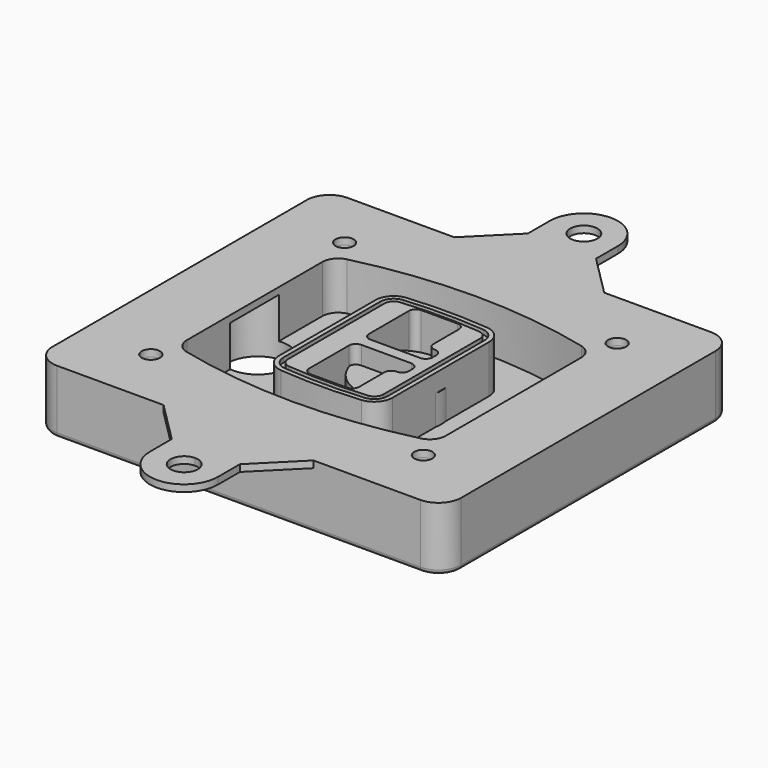
from build123d import *

# Parameters (mm, degrees)
F0_R      = 4
F1_DEPTH  = 25
F2_DEPTH  = 3
F3_DEPTH  = 18
F5_DEPTH  = 21
F6_DEPTH  = 2
F8_DEPTH  = 20
F9_DEPTH  = 16
F10_DEPTH = 25
F7_R      = 6
F7_R_2    = 4
F11_DEPTH = 6
F13_DEPTH = 9
F15_R     = 2
F16_R     = 4
F17_DEPTH = 3


# Not quite as in the source:
# - a feature of the source that left no trace in its solid (it failed there, or was rolled back) is left out
# - a feature names something its author has since deleted; it is built from what else it names


with BuildPart() as f1:
    # F0 (on Top) → F1 (new body)
    with BuildSketch(Plane.XY):
        with BuildLine():
            ThreePointArc((-90, -70), (-87.0710678119, -77.0710678119), (-80, -80))
            Line((-80, -80), (80, -80))
            ThreePointArc((80, -80), (87.0710678119, -77.0710678119), (90, -70))
            Line((90, -70), (90, 70))
            ThreePointArc((90, 70), (87.0710678119, 77.0710678119), (80, 80))
            Line((80, 80), (-80, 80))
            ThreePointArc((-80, 80), (-87.0710678119, 77.0710678119), (-90, 70))
            Line((-90, 70), (-90, -70))
        make_face()
        with Locations((-60, -53.3333333333)):
            Circle(F0_R, mode=Mode.SUBTRACT)
        with Locations((60, -53.3333333333)):
            Circle(F0_R, mode=Mode.SUBTRACT)
        with Locations((-60, 53.3333333333)):
            Circle(F0_R, mode=Mode.SUBTRACT)
        with BuildLine():
            ThreePointArc((-64, 37.2990447398), (-61.0143011354, 45.9411029726), (-53.3306899286, 50.8970778549))
            ThreePointArc((-53.3306899286, 50.8970778549), (0, 57.3333333333), (53.3306899286, 50.8970778549))
            ThreePointArc((53.3306899286, 50.8970778549), (61.0143011354, 45.9411029726), (64, 37.2990447398))
            Line((64, 37.2990447398), (64, -37.2990447398))
            ThreePointArc((64, -37.2990447398), (61.0143011354, -45.9411029726), (53.3306899286, -50.8970778549))
            ThreePointArc((53.3306899286, -50.8970778549), (0, -57.3333333333), (-53.3306899286, -50.8970778549))
            ThreePointArc((-53.3306899286, -50.8970778549), (-61.0143011354, -45.9411029726), (-64, -37.2990447398))
            Line((-64, -37.2990447398), (-64, 37.2990447398))
        make_face(mode=Mode.SUBTRACT)
        with Locations((60, 53.3333333333)):
            Circle(F0_R, mode=Mode.SUBTRACT)
        with BuildLine():
            ThreePointArc((53.3306899286, 50.8970778549), (0, 57.3333333333), (-53.3306899286, 50.8970778549))
            ThreePointArc((-53.3306899286, 50.8970778549), (-61.0143011354, 45.9411029726), (-64, 37.2990447398))
            Line((-64, 37.2990447398), (-64, -37.2990447398))
            ThreePointArc((-64, -37.2990447398), (-61.0143011354, -45.9411029726), (-53.3306899286, -50.8970778549))
            ThreePointArc((-53.3306899286, -50.8970778549), (0, -57.3333333333), (53.3306899286, -50.8970778549))
            ThreePointArc((53.3306899286, -50.8970778549), (61.0143011354, -45.9411029726), (64, -37.2990447398))
            Line((64, -37.2990447398), (64, 37.2990447398))
            ThreePointArc((64, 37.2990447398), (61.0143011354, 45.9411029726), (53.3306899286, 50.8970778549))
        make_face()
        with BuildLine():
            Line((-60, -37.2990447398), (-60, 37.2990447398))
            ThreePointArc((-60, 37.2990447398), (-57.8673579538, 43.4719434775), (-52.3790642347, 47.0119255363))
            ThreePointArc((-52.3790642347, 47.0119255363), (0, 53.3333333333), (52.3790642347, 47.0119255363))
            ThreePointArc((52.3790642347, 47.0119255363), (57.8673579538, 43.4719434775), (60, 37.2990447398))
            Line((60, 37.2990447398), (60, -37.2990447398))
            ThreePointArc((60, -37.2990447398), (57.8673579538, -43.4719434775), (52.3790642347, -47.0119255363))
            ThreePointArc((52.3790642347, -47.0119255363), (0, -53.3333333333), (-52.3790642347, -47.0119255363))
            ThreePointArc((-52.3790642347, -47.0119255363), (-57.8673579538, -43.4719434775), (-60, -37.2990447398))
        make_face(mode=Mode.SUBTRACT)
        with BuildLine():
            ThreePointArc((-52.3790642347, 47.0119255363), (-57.8673579538, 43.4719434775), (-60, 37.2990447398))
            Line((-60, 37.2990447398), (-60, -37.2990447398))
            ThreePointArc((-60, -37.2990447398), (-57.8673579538, -43.4719434775), (-52.3790642347, -47.0119255363))
            ThreePointArc((-52.3790642347, -47.0119255363), (0, -53.3333333333), (52.3790642347, -47.0119255363))
            ThreePointArc((52.3790642347, -47.0119255363), (57.8673579538, -43.4719434775), (60, -37.2990447398))
            Line((60, -37.2990447398), (60, 37.2990447398))
            ThreePointArc((60, 37.2990447398), (57.8673579538, 43.4719434775), (52.3790642347, 47.0119255363))
            ThreePointArc((52.3790642347, 47.0119255363), (0, 53.3333333333), (-52.3790642347, 47.0119255363))
        make_face()
        with BuildLine():
            ThreePointArc((51.6653449643, 44.0980612973), (55.5071505677, 41.6200738562), (57, 37.2990447398))
            Line((57, 37.2990447398), (57, -37.2990447398))
            ThreePointArc((57, -37.2990447398), (55.5071505677, -41.6200738562), (51.6653449643, -44.0980612973))
            ThreePointArc((51.6653449643, -44.0980612973), (0, -50.3333333333), (-51.6653449643, -44.0980612973))
            ThreePointArc((-51.6653449643, -44.0980612973), (-55.5071505677, -41.6200738562), (-57, -37.2990447398))
            Line((-57, -37.2990447398), (-57, 37.2990447398))
            ThreePointArc((-57, 37.2990447398), (-55.5071505677, 41.6200738562), (-51.6653449643, 44.0980612973))
            ThreePointArc((-51.6653449643, 44.0980612973), (0, 50.3333333333), (51.6653449643, 44.0980612973))
        make_face(mode=Mode.SUBTRACT)
        with BuildLine():
            Line((57, -37.2990447398), (57, 37.2990447398))
            ThreePointArc((57, 37.2990447398), (55.5071505677, 41.6200738562), (51.6653449643, 44.0980612973))
            ThreePointArc((51.6653449643, 44.0980612973), (0, 50.3333333333), (-51.6653449643, 44.0980612973))
            ThreePointArc((-51.6653449643, 44.0980612973), (-55.5071505677, 41.6200738562), (-57, 37.2990447398))
            Line((-57, 37.2990447398), (-57, -37.2990447398))
            ThreePointArc((-57, -37.2990447398), (-55.5071505677, -41.6200738562), (-51.6653449643, -44.0980612973))
            ThreePointArc((-51.6653449643, -44.0980612973), (0, -50.3333333333), (51.6653449643, -44.0980612973))
            ThreePointArc((51.6653449643, -44.0980612973), (55.5071505677, -41.6200738562), (57, -37.2990447398))
        make_face()
    extrude(amount=-F1_DEPTH)

    # F0 (on Top) → F2 (join)
    with BuildSketch(Plane.XY):
        with BuildLine():
            ThreePointArc((-52.3790642347, 47.0119255363), (-57.8673579538, 43.4719434775), (-60, 37.2990447398))
            Line((-60, 37.2990447398), (-60, -37.2990447398))
            ThreePointArc((-60, -37.2990447398), (-57.8673579538, -43.4719434775), (-52.3790642347, -47.0119255363))
            ThreePointArc((-52.3790642347, -47.0119255363), (0, -53.3333333333), (52.3790642347, -47.0119255363))
            ThreePointArc((52.3790642347, -47.0119255363), (57.8673579538, -43.4719434775), (60, -37.2990447398))
            Line((60, -37.2990447398), (60, 37.2990447398))
            ThreePointArc((60, 37.2990447398), (57.8673579538, 43.4719434775), (52.3790642347, 47.0119255363))
            ThreePointArc((52.3790642347, 47.0119255363), (0, 53.3333333333), (-52.3790642347, 47.0119255363))
        make_face()
        with BuildLine():
            ThreePointArc((51.6653449643, 44.0980612973), (55.5071505677, 41.6200738562), (57, 37.2990447398))
            Line((57, 37.2990447398), (57, -37.2990447398))
            ThreePointArc((57, -37.2990447398), (55.5071505677, -41.6200738562), (51.6653449643, -44.0980612973))
            ThreePointArc((51.6653449643, -44.0980612973), (0, -50.3333333333), (-51.6653449643, -44.0980612973))
            ThreePointArc((-51.6653449643, -44.0980612973), (-55.5071505677, -41.6200738562), (-57, -37.2990447398))
            Line((-57, -37.2990447398), (-57, 37.2990447398))
            ThreePointArc((-57, 37.2990447398), (-55.5071505677, 41.6200738562), (-51.6653449643, 44.0980612973))
            ThreePointArc((-51.6653449643, 44.0980612973), (0, 50.3333333333), (51.6653449643, 44.0980612973))
        make_face(mode=Mode.SUBTRACT)
    extrude(amount=F2_DEPTH)

    # F0 (on Top) → F3 (cut)
    with BuildSketch(Plane.XY):
        with BuildLine():
            Line((57, -37.2990447398), (57, 37.2990447398))
            ThreePointArc((57, 37.2990447398), (55.5071505677, 41.6200738562), (51.6653449643, 44.0980612973))
            ThreePointArc((51.6653449643, 44.0980612973), (0, 50.3333333333), (-51.6653449643, 44.0980612973))
            ThreePointArc((-51.6653449643, 44.0980612973), (-55.5071505677, 41.6200738562), (-57, 37.2990447398))
            Line((-57, 37.2990447398), (-57, -37.2990447398))
            ThreePointArc((-57, -37.2990447398), (-55.5071505677, -41.6200738562), (-51.6653449643, -44.0980612973))
            ThreePointArc((-51.6653449643, -44.0980612973), (0, -50.3333333333), (51.6653449643, -44.0980612973))
            ThreePointArc((51.6653449643, -44.0980612973), (55.5071505677, -41.6200738562), (57, -37.2990447398))
        make_face()
    extrude(amount=-F3_DEPTH, mode=Mode.SUBTRACT)

    # F4 (on face) → F5 (join, through all)
    with BuildSketch(Plane.XY.offset(3)):
        with BuildLine():
            ThreePointArc((-25, -26.587695628), (-22.8992979869, -31.9912392117), (-17.7004291845, -34.5569740744))
            ThreePointArc((-17.7004291845, -34.5569740744), (0, -35.3333333333), (17.7004291845, -34.5569740744))
            ThreePointArc((17.7004291845, -34.5569740744), (22.8992979869, -31.9912392117), (25, -26.587695628))
            Line((25, -26.587695628), (25, 26.587695628))
            ThreePointArc((25, 26.587695628), (22.8992979869, 31.9912392117), (17.7004291845, 34.5569740744))
            ThreePointArc((17.7004291845, 34.5569740744), (0, 35.3333333333), (-17.7004291845, 34.5569740744))
            ThreePointArc((-17.7004291845, 34.5569740744), (-22.8992979869, 31.9912392117), (-25, 26.587695628))
            Line((-25, 26.587695628), (-25, -26.587695628))
        make_face()
        with BuildLine():
            ThreePointArc((17.5253218884, 32.5646544628), (21.4244734902, 30.6403533158), (23, 26.587695628))
            Line((23, 26.587695628), (23, -26.587695628))
            ThreePointArc((23, -26.587695628), (21.4244734902, -30.6403533158), (17.5253218884, -32.5646544628))
            ThreePointArc((17.5253218884, -32.5646544628), (0, -33.3333333333), (-17.5253218884, -32.5646544628))
            ThreePointArc((-17.5253218884, -32.5646544628), (-21.4244734902, -30.6403533158), (-23, -26.587695628))
            Line((-23, -26.587695628), (-23, 26.587695628))
            ThreePointArc((-23, 26.587695628), (-21.4244734902, 30.6403533158), (-17.5253218884, 32.5646544628))
            ThreePointArc((-17.5253218884, 32.5646544628), (0, 33.3333333333), (17.5253218884, 32.5646544628))
        make_face(mode=Mode.SUBTRACT)
        with BuildLine():
            Line((23, -26.587695628), (23, 26.587695628))
            ThreePointArc((23, 26.587695628), (21.4244734902, 30.6403533158), (17.5253218884, 32.5646544628))
            ThreePointArc((17.5253218884, 32.5646544628), (0, 33.3333333333), (-17.5253218884, 32.5646544628))
            ThreePointArc((-17.5253218884, 32.5646544628), (-21.4244734902, 30.6403533158), (-23, 26.587695628))
            Line((-23, 26.587695628), (-23, -26.587695628))
            ThreePointArc((-23, -26.587695628), (-21.4244734902, -30.6403533158), (-17.5253218884, -32.5646544628))
            ThreePointArc((-17.5253218884, -32.5646544628), (0, -33.3333333333), (17.5253218884, -32.5646544628))
            ThreePointArc((17.5253218884, -32.5646544628), (21.4244734902, -30.6403533158), (23, -26.587695628))
        make_face()
        with BuildLine():
            ThreePointArc((17.3502145923, 30.5723348512), (19.9496489934, 29.2894674198), (21, 26.587695628))
            Line((21, 26.587695628), (21, -26.587695628))
            ThreePointArc((21, -26.587695628), (19.9496489934, -29.2894674198), (17.3502145923, -30.5723348512))
            ThreePointArc((17.3502145923, -30.5723348512), (0, -31.3333333333), (-17.3502145923, -30.5723348512))
            ThreePointArc((-17.3502145923, -30.5723348512), (-19.9496489934, -29.2894674198), (-21, -26.587695628))
            Line((-21, -26.587695628), (-21, 26.587695628))
            ThreePointArc((-21, 26.587695628), (-19.9496489934, 29.2894674198), (-17.3502145923, 30.5723348512))
            ThreePointArc((-17.3502145923, 30.5723348512), (0, 31.3333333333), (17.3502145923, 30.5723348512))
        make_face(mode=Mode.SUBTRACT)
        with BuildLine():
            Line((21, -26.587695628), (21, 26.587695628))
            ThreePointArc((21, 26.587695628), (19.9496489934, 29.2894674198), (17.3502145923, 30.5723348512))
            ThreePointArc((17.3502145923, 30.5723348512), (0, 31.3333333333), (-17.3502145923, 30.5723348512))
            ThreePointArc((-17.3502145923, 30.5723348512), (-19.9496489934, 29.2894674198), (-21, 26.587695628))
            Line((-21, 26.587695628), (-21, -26.587695628))
            ThreePointArc((-21, -26.587695628), (-19.9496489934, -29.2894674198), (-17.3502145923, -30.5723348512))
            ThreePointArc((-17.3502145923, -30.5723348512), (0, -31.3333333333), (17.3502145923, -30.5723348512))
            ThreePointArc((17.3502145923, -30.5723348512), (19.9496489934, -29.2894674198), (21, -26.587695628))
        make_face()
        with BuildLine():
            Line((-8, -2.5), (14, -2.5))
            ThreePointArc((14, -2.5), (16.1213203436, -3.3786796564), (17, -5.5))
            Line((17, -5.5), (17, -7.5))
            ThreePointArc((17, -7.5), (16.1213203436, -9.6213203436), (14, -10.5))
            ThreePointArc((14, -10.5), (11.8786796564, -11.3786796564), (11, -13.5))
            Line((11, -13.5), (11, -27.5))
            ThreePointArc((11, -27.5), (10.1213203436, -29.6213203436), (8, -30.5))
            Line((8, -30.5), (-8, -30.5))
            ThreePointArc((-8, -30.5), (-10.1213203436, -29.6213203436), (-11, -27.5))
            Line((-11, -27.5), (-11, -5.5))
            ThreePointArc((-11, -5.5), (-10.1213203436, -3.3786796564), (-8, -2.5))
        make_face(mode=Mode.SUBTRACT)
        with BuildLine():
            ThreePointArc((-8, 2.5), (-10.1213203436, 3.3786796564), (-11, 5.5))
            Line((-11, 5.5), (-11, 27.5))
            ThreePointArc((-11, 27.5), (-10.1213203436, 29.6213203436), (-8, 30.5))
            Line((-8, 30.5), (8, 30.5))
            ThreePointArc((8, 30.5), (10.1213203436, 29.6213203436), (11, 27.5))
            Line((11, 27.5), (11, 13.5))
            ThreePointArc((11, 13.5), (11.8786796564, 11.3786796564), (14, 10.5))
            ThreePointArc((14, 10.5), (16.1213203436, 9.6213203436), (17, 7.5))
            Line((17, 7.5), (17, 5.5))
            ThreePointArc((17, 5.5), (16.1213203436, 3.3786796564), (14, 2.5))
            Line((14, 2.5), (-8, 2.5))
        make_face(mode=Mode.SUBTRACT)
    extrude(amount=-F5_DEPTH)

    # F4 (on face) → F6 (cut)
    with BuildSketch(Plane.XY.offset(3)):
        with BuildLine():
            Line((23, -26.587695628), (23, 26.587695628))
            ThreePointArc((23, 26.587695628), (21.4244734902, 30.6403533158), (17.5253218884, 32.5646544628))
            ThreePointArc((17.5253218884, 32.5646544628), (0, 33.3333333333), (-17.5253218884, 32.5646544628))
            ThreePointArc((-17.5253218884, 32.5646544628), (-21.4244734902, 30.6403533158), (-23, 26.587695628))
            Line((-23, 26.587695628), (-23, -26.587695628))
            ThreePointArc((-23, -26.587695628), (-21.4244734902, -30.6403533158), (-17.5253218884, -32.5646544628))
            ThreePointArc((-17.5253218884, -32.5646544628), (0, -33.3333333333), (17.5253218884, -32.5646544628))
            ThreePointArc((17.5253218884, -32.5646544628), (21.4244734902, -30.6403533158), (23, -26.587695628))
        make_face()
        with BuildLine():
            ThreePointArc((17.3502145923, 30.5723348512), (19.9496489934, 29.2894674198), (21, 26.587695628))
            Line((21, 26.587695628), (21, -26.587695628))
            ThreePointArc((21, -26.587695628), (19.9496489934, -29.2894674198), (17.3502145923, -30.5723348512))
            ThreePointArc((17.3502145923, -30.5723348512), (0, -31.3333333333), (-17.3502145923, -30.5723348512))
            ThreePointArc((-17.3502145923, -30.5723348512), (-19.9496489934, -29.2894674198), (-21, -26.587695628))
            Line((-21, -26.587695628), (-21, 26.587695628))
            ThreePointArc((-21, 26.587695628), (-19.9496489934, 29.2894674198), (-17.3502145923, 30.5723348512))
            ThreePointArc((-17.3502145923, 30.5723348512), (0, 31.3333333333), (17.3502145923, 30.5723348512))
        make_face(mode=Mode.SUBTRACT)
    extrude(amount=-F6_DEPTH, mode=Mode.SUBTRACT)

    # F7 (on face) → F8 (join)
    with BuildSketch(Plane(origin=(0, 0, -25), x_dir=(1, 0, 0), z_dir=(0, 0, -1))):
        with BuildLine():
            ThreePointArc((-6.71157564, 0), (6.7567035675, 13.4682792075), (20.224982775, 0))
            Line((20.224982775, 0), (25.224982775, 0))
            ThreePointArc((25.224982775, 0), (6.7567035675, 18.4682792075), (-11.71157564, 0))
            Line((-11.71157564, 0), (-6.71157564, 0))
        make_face()
        with BuildLine():
            Line((-6.71157564, 0), (20.224982775, 0))
            ThreePointArc((20.224982775, 0), (6.7567035675, 13.4682792075), (-6.71157564, 0))
        make_face()
        with BuildLine():
            ThreePointArc((-6.71157564, 0), (6.7567035675, -13.4682792075), (20.224982775, 0))
            Line((20.224982775, 0), (-6.71157564, 0))
        make_face()
        with BuildLine():
            Line((25.224982775, 0), (20.224982775, 0))
            ThreePointArc((20.224982775, 0), (6.7567035675, -13.4682792075), (-6.71157564, 0))
            Line((-6.71157564, 0), (-11.71157564, 0))
            ThreePointArc((-11.71157564, 0), (6.7567035675, -18.4682792075), (25.224982775, 0))
        make_face()
    extrude(amount=-F8_DEPTH)

    # F7 (on face) → F9 (cut)
    with BuildSketch(Plane(origin=(0, 0, -25), x_dir=(1, 0, 0), z_dir=(0, 0, -1))):
        with BuildLine():
            Line((-6.71157564, 0), (20.224982775, 0))
            ThreePointArc((20.224982775, 0), (6.7567035675, 13.4682792075), (-6.71157564, 0))
        make_face()
        with BuildLine():
            ThreePointArc((-6.71157564, 0), (6.7567035675, -13.4682792075), (20.224982775, 0))
            Line((20.224982775, 0), (-6.71157564, 0))
        make_face()
    extrude(amount=-F9_DEPTH, mode=Mode.SUBTRACT)

    # F7 (on face) → F10 (cut)
    with BuildSketch(Plane(origin=(0, 0, -25), x_dir=(1, 0, 0), z_dir=(0, 0, -1))):
        with BuildLine():
            Line((-69.0318229325, 0), (-42.0952645175, 0))
            ThreePointArc((-42.0952645175, 0), (-55.563543725, 13.4682792075), (-69.0318229325, 0))
        make_face()
        with BuildLine():
            ThreePointArc((-69.0318229325, 0), (-55.563543725, -13.4682792075), (-42.0952645175, 0))
            Line((-42.0952645175, 0), (-69.0318229325, 0))
        make_face()
    extrude(amount=-F10_DEPTH, mode=Mode.SUBTRACT)

    # F7 (on face) → F11 (cut)
    with BuildSketch(Plane(origin=(0, 0, -25), x_dir=(1, 0, 0), z_dir=(0, 0, -1))):
        with Locations((60, -53.3333333333)):
            Circle(F7_R)
        with Locations((60, -53.3333333333)):
            Circle(F7_R_2, mode=Mode.SUBTRACT)
        with Locations((-60, -53.3333333333)):
            Circle(F7_R)
        with Locations((-60, -53.3333333333)):
            Circle(F7_R_2, mode=Mode.SUBTRACT)
        with Locations((-60, 53.3333333333)):
            Circle(F7_R)
        with Locations((-60, 53.3333333333)):
            Circle(F7_R_2, mode=Mode.SUBTRACT)
        with Locations((60, 53.3333333333)):
            Circle(F7_R)
        with Locations((60, 53.3333333333)):
            Circle(F7_R_2, mode=Mode.SUBTRACT)
    extrude(amount=-F11_DEPTH, mode=Mode.SUBTRACT)

    # F12 (on face) → F13 (cut, through all)
    with BuildSketch(Plane(origin=(0, 0, -9), x_dir=(1, 0, 0), z_dir=(0, 0, -1))):
        with BuildLine():
            ThreePointArc((20.224982775, 0), (20.1663399806, 1.2554664788), (19.9909222755, 2.5))
            Line((19.9909222755, 2.5), (14, 2.5))
            ThreePointArc((14, 2.5), (16.1213203436, 3.3786796564), (17, 5.5))
            Line((17, 5.5), (17, 7.5))
            ThreePointArc((17, 7.5), (16.1213203436, 9.6213203436), (14, 10.5))
            ThreePointArc((14, 10.5), (12.1627255951, 11.1284134507), (11.0951631559, 12.750384826))
            ThreePointArc((11.0951631559, 12.750384826), (11.0476113807, 12.7664660322), (11, 12.7823698976))
            Line((11, 12.7823698976), (11, -12.7823698976))
            ThreePointArc((11, -12.7823698976), (11.0476113807, -12.7664660322), (11.0951631559, -12.750384826))
            ThreePointArc((11.0951631559, -12.750384826), (12.1627255951, -11.1284134507), (14, -10.5))
            ThreePointArc((14, -10.5), (16.1213203436, -9.6213203436), (17, -7.5))
            Line((17, -7.5), (17, -5.5))
            ThreePointArc((17, -5.5), (16.1213203436, -3.3786796564), (14, -2.5))
            Line((14, -2.5), (19.9909222755, -2.5))
            ThreePointArc((19.9909222755, -2.5), (20.1663399806, -1.2554664788), (20.224982775, 0))
        make_face()
    extrude(amount=F13_DEPTH, mode=Mode.SUBTRACT)

    # F15
    f15_edges = [f1.edges().sort_by_distance(p)[0] for p in [
        (0, -80, -25),
        (-87.071068, -77.071068, -25),
        (-90, 0, -25),
        (-87.071068, 77.071068, -25),
        (87.071068, -77.071068, -25),
        (0, 80, -25),
        (90, 0, -25),
        (87.071068, 77.071068, -25),
    ]]
    fillet(f15_edges, radius=F15_R)

    # F16 (on face) → F17 (join, through all)
    with BuildSketch(Plane.XY):
        with BuildLine():
            Line((-90, 70), (-90, -70))
            ThreePointArc((-90, -70), (-87.0710678119, -77.0710678119), (-80, -80))
            Line((-80, -80), (-33.0487348606, -80))
            Line((-33.0487348606, -80), (0, -80))
            Line((0, -80), (32.9512651394, -80))
            Line((32.9512651394, -80), (80, -80))
            ThreePointArc((80, -80), (87.0710678119, -77.0710678119), (90, -70))
            Line((90, -70), (90, 70))
            ThreePointArc((90, 70), (87.0710678119, 77.0710678119), (80, 80))
            Line((80, 80), (32.9512651394, 80))
            Line((32.9512651394, 80), (0, 80))
            Line((0, 80), (-33.0487348606, 80))
            Line((-33.0487348606, 80), (-80, 80))
            ThreePointArc((-80, 80), (-87.0710678119, 77.0710678119), (-90, 70))
        make_face()
        with Locations((-60, -53.3333333333)):
            Circle(F16_R, mode=Mode.SUBTRACT)
        with Locations((60, -53.3333333333)):
            Circle(F16_R, mode=Mode.SUBTRACT)
        with Locations((-60, 53.3333333333)):
            Circle(F16_R, mode=Mode.SUBTRACT)
        with BuildLine():
            Line((-60, -37.2990447398), (-60, 37.2990447398))
            ThreePointArc((-60, 37.2990447398), (-57.8673579538, 43.4719434775), (-52.3790642347, 47.0119255363))
            ThreePointArc((-52.3790642347, 47.0119255363), (0, 53.3333333333), (52.3790642347, 47.0119255363))
            ThreePointArc((52.3790642347, 47.0119255363), (57.8673579538, 43.4719434775), (60, 37.2990447398))
            Line((60, 37.2990447398), (60, -37.2990447398))
            ThreePointArc((60, -37.2990447398), (57.8673579538, -43.4719434775), (52.3790642347, -47.0119255363))
            ThreePointArc((52.3790642347, -47.0119255363), (0, -53.3333333333), (-52.3790642347, -47.0119255363))
            ThreePointArc((-52.3790642347, -47.0119255363), (-57.8673579538, -43.4719434775), (-60, -37.2990447398))
        make_face(mode=Mode.SUBTRACT)
        with Locations((60, 53.3333333333)):
            Circle(F16_R, mode=Mode.SUBTRACT)
        with BuildLine():
            Line((0, -80), (-33.0487348606, -80))
            Line((-33.0487348606, -80), (-15.0487348606, -98))
            Line((-15.0487348606, -98), (-15.0487348606, -110))
            ThreePointArc((-15.0487348606, -110), (-0.0487348606, -125), (14.9512651394, -110))
            Line((14.9512651394, -110), (14.9512651394, -98))
            Line((14.9512651394, -98), (32.9512651394, -80))
            Line((32.9512651394, -80), (0, -80))
        make_face()
        with BuildLine():
            ThreePointArc((6, -110), (-4.2426406871, -114.2426406871), (0, -104))
            ThreePointArc((0, -104), (4.2426406871, -105.7573593129), (6, -110))
        make_face(mode=Mode.SUBTRACT)
        with BuildLine():
            Line((-15.0487348606, 98), (-33.0487348606, 80))
            Line((-33.0487348606, 80), (0, 80))
            Line((0, 80), (32.9512651394, 80))
            Line((32.9512651394, 80), (14.9512651394, 98))
            Line((14.9512651394, 98), (14.9512651394, 110))
            ThreePointArc((14.9512651394, 110), (-0.0487348606, 125), (-15.0487348606, 110))
            Line((-15.0487348606, 110), (-15.0487348606, 98))
        make_face()
        with BuildLine():
            ThreePointArc((6, 110), (4.2426406871, 105.7573593129), (0, 104))
            ThreePointArc((0, 104), (-4.2426406871, 114.2426406871), (6, 110))
        make_face(mode=Mode.SUBTRACT)
    extrude(amount=F17_DEPTH)


solid = f1.part
